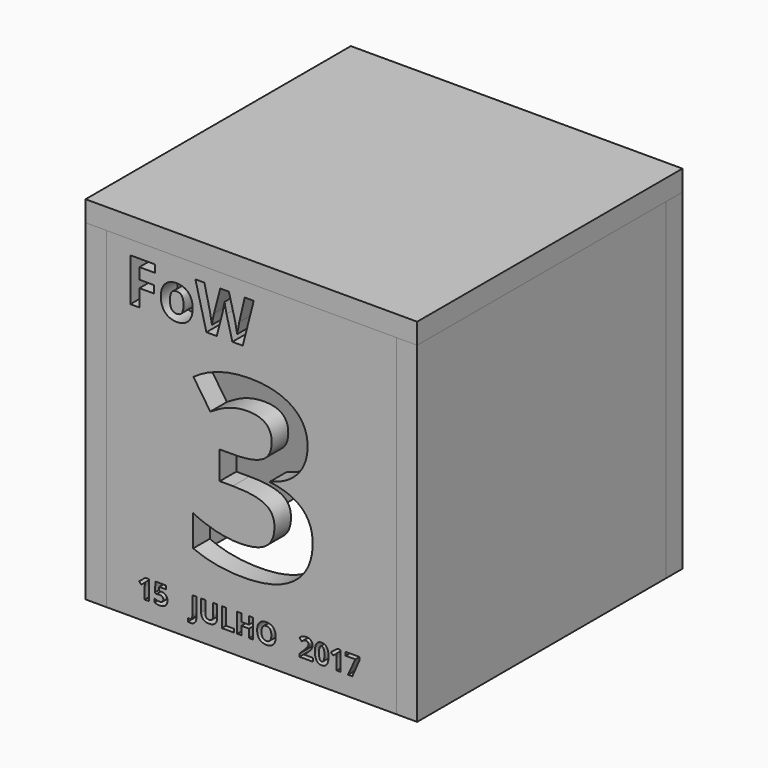
from build123d import *

# Parameters (mm, degrees)
F0_W            = 40
F0_H            = 40
F1_DEPTH        = 2.5
F2_W            = 40
F2_H            = 40
F3_DEPTH        = 2.5
F4_W            = 40
F4_H            = 40
F5_DEPTH        = 2.5
F6_W            = 40
F6_H            = 40
F7_DEPTH        = 2.5
F8_W            = 40
F8_H            = 40
F9_DEPTH        = 2.5
F10_TEXT_SIZE   = 7.2732438383
F10_TEXT_SIZE_2 = 29.1666666667
F10_TEXT_SIZE_3 = 3.2806804374
F11_DEPTH       = 3


# Not quite as in the source:
# - Text() gives the source's letters only with a copy of the font that has no kerning and outlines rounded to 1/6400 em; it was checked with that copy


with BuildPart() as f1:
    # F0 (on Top) → F1 (new body)
    with BuildSketch(Plane.XY):
        with Locations((-20, 20)):
            Rectangle(F0_W, F0_H)
    extrude(amount=F1_DEPTH)


with BuildPart() as f3:
    # F2 (on face) → F3 (new body)
    with BuildSketch(Plane.XZ):
        with Locations((-20, -20)):
            Rectangle(F2_W, F2_H)
    extrude(amount=-F3_DEPTH)

    # F10 (on face) → F11 (cut)
    with BuildSketch(Plane.XZ):
        with Locations((-35.2436941774, -6.8869412126)):
            Text('FoW', F10_TEXT_SIZE, font='Open Sans', font_style=FontStyle.BOLD, text_align=(TextAlign.LEFT, TextAlign.BOTTOM))
        with Locations((-28.1307792269, -31.1978415623)):
            Text('3', F10_TEXT_SIZE_2, font='Open Sans', font_style=FontStyle.BOLD, text_align=(TextAlign.LEFT, TextAlign.BOTTOM))
        with Locations((-33.7231783196, -37.6993305981)):
            Text('15   JULHO   2017', F10_TEXT_SIZE_3, font='Open Sans', font_style=FontStyle.BOLD, text_align=(TextAlign.LEFT, TextAlign.BOTTOM))
    extrude(amount=-F11_DEPTH, mode=Mode.SUBTRACT)


with BuildPart() as f5:
    # F4 (on face) → F5 (new body)
    with BuildSketch(Plane.YZ):
        with Locations((20, -20)):
            Rectangle(F4_W, F4_H)
    extrude(amount=-F5_DEPTH)


with BuildPart() as f7:
    # F6 (on face) → F7 (new body)
    with BuildSketch(Plane(origin=(0, 40, 0), x_dir=(-1, 0, 0), z_dir=(0, 1, 0))):
        with Locations((20, -20)):
            Rectangle(F6_W, F6_H)
    extrude(amount=-F7_DEPTH)


with BuildPart() as f9:
    # F8 (on face) → F9 (new body)
    with BuildSketch(Plane(origin=(-40, 0, 0), x_dir=(0, -1, 0), z_dir=(-1, 0, 0))):
        with Locations((-20, -20)):
            Rectangle(F8_W, F8_H)
    extrude(amount=-F9_DEPTH)


solid = Compound([f1.part, f3.part, f5.part, f7.part, f9.part])
